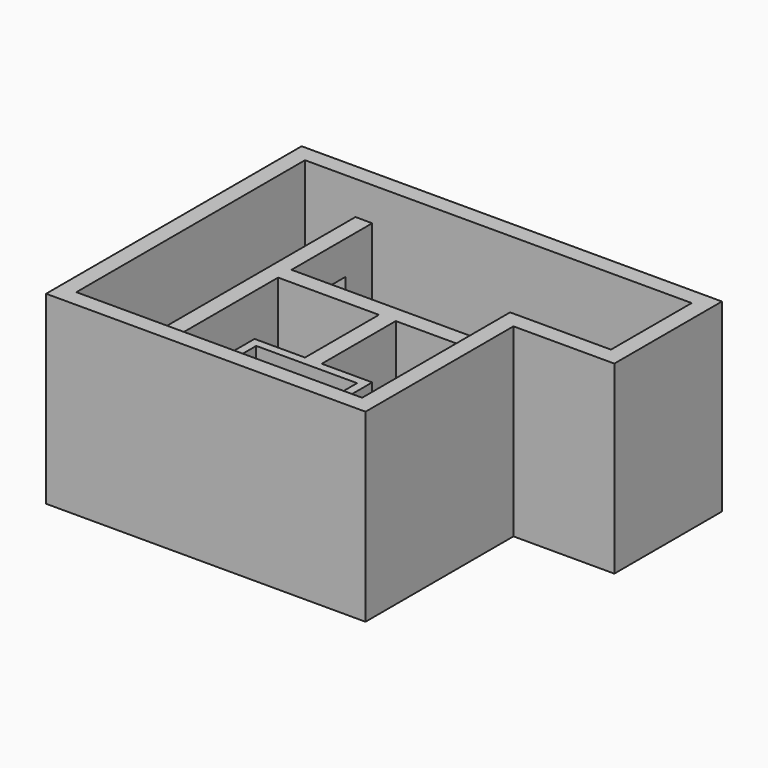
from build123d import *

# Parameters (mm, degrees)
F1_DEPTH = 25.4
F3_DEPTH = 254
F4_W     = 25.4
F4_H     = 139.7
F4_H_2   = 25.4
F4_H_3   = 12.7
F4_W_2   = 63.5
F4_W_3   = 12.7
F4_H_4   = 254
F4_H_5   = 152.4
F4_H_6   = 101.6
F5_DEPTH = 203.2
F6_W     = 25.4
F6_H     = 76.2
F7_DEPTH = 101.6
F8_W     = 50.8
F8_H     = 152.4
F9_DEPTH = 25.4


with BuildPart() as f1:
    # F0 (on Top) → F1 (new body)
    with BuildSketch(Plane.XY):
        Polygon((-482.6, 0), (0, 0), (0, 279.4), (152.4, 279.4), (152.4, 482.6), (-482.6, 482.6), align=None)
    extrude(amount=F1_DEPTH)

    # F2 (on face) → F3 (join)
    with BuildSketch(Plane.XY.offset(25.4)):
        Polygon((152.4, 279.4), (152.4, 482.6), (-482.6, 482.6), (-482.6, 0), (0, 0), (0, 279.4), align=None)
        Polygon((-25.4, 25.4), (-457.2, 25.4), (-457.2, 457.2), (127, 457.2), (127, 304.8), (-25.4, 304.8), align=None, mode=Mode.SUBTRACT)
    extrude(amount=F3_DEPTH)

    # F4 (on face) → F5 (join)
    with BuildSketch(Plane.XY.offset(25.4)):
        with Locations((-190.5, 209.55)):
            Rectangle(F4_W, F4_H)
        with Locations((-368.3, 292.1)):
            Rectangle(F4_W, F4_H_2)
        with Locations((-190.5, 133.35)):
            Rectangle(F4_W, F4_H_3)
        with Locations((-234.95, 133.35)):
            Rectangle(F4_W_2, F4_H_3)
        with Locations((-146.05, 133.35)):
            Rectangle(F4_W_2, F4_H_3)
        with Locations((-273.05, 133.35)):
            Rectangle(F4_W_3, F4_H_3)
        with Locations((-107.95, 133.35)):
            Rectangle(F4_W_3, F4_H_3)
        with Locations((-368.3, 152.4)):
            Rectangle(F4_W, F4_H_4)
        Polygon((-355.6, 304.8), (-355.6, 279.4), (-203.2, 279.4), (-177.8, 279.4), (-25.4, 279.4), (-25.4, 304.8), align=None)
        with Locations((-368.3, 381)):
            Rectangle(F4_W, F4_H_5)
        with Locations((-107.95, 76.2)):
            Rectangle(F4_W_3, F4_H_6)
        with Locations((-273.05, 76.2)):
            Rectangle(F4_W_3, F4_H_6)
    extrude(amount=F5_DEPTH)

    # F6 (on face) → F7 (join)
    with BuildSketch(Plane.XY.offset(25.4)):
        with Locations((-9.9159989834, 342.9)):
            Rectangle(F6_W, F6_H)
    extrude(amount=F7_DEPTH)

    # F8 (on face) → F9 (cut)
    with BuildSketch(Plane.YZ.offset(-355.6)):
        with Locations((381, 101.6)):
            Rectangle(F8_W, F8_H)
    extrude(amount=-F9_DEPTH, mode=Mode.SUBTRACT)


solid = f1.part
